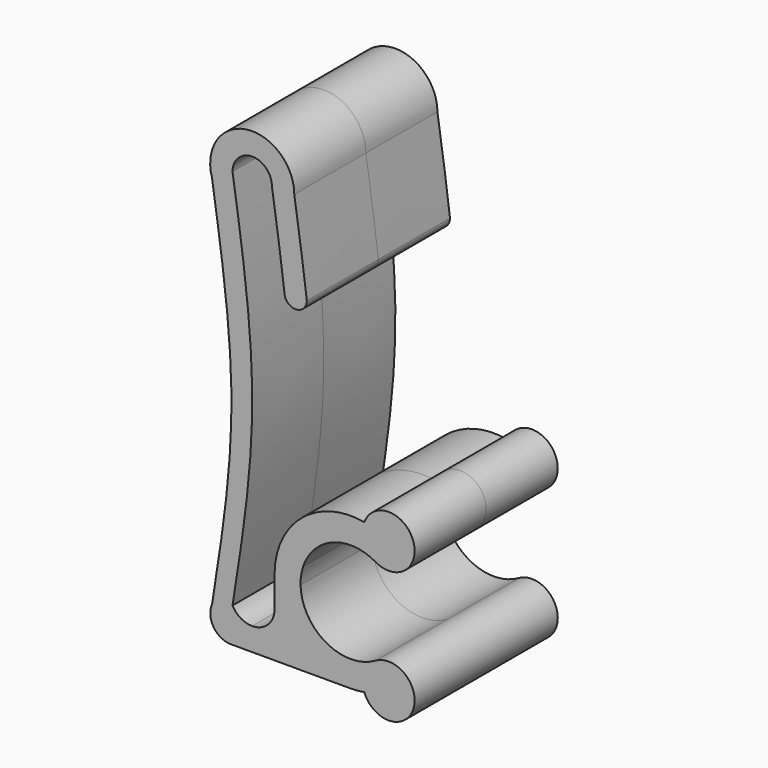
from build123d import *

# Parameters (mm, degrees)
F1_DEPTH = 6.35


# Not quite as in the source:
# - ends of sketch curves that miss each other by under 0.0002 mm in the source are joined
# - the dataset's text gives a spline's control points without its knots; the knots are read off the source's solid


with BuildPart() as f1:
    # F0 (on Front) → F1 (new body, symmetric)
    with BuildSketch(Plane.XZ):
        with BuildLine():
            Line((-8.4141566916, -5.3975), (0, -5.3975))
            ThreePointArc((0, -5.3975), (0.4871232852, -5.375473668), (0.9702708263, -5.3095744437))
            ThreePointArc((0.9702708263, -5.3095744437), (4.4301700946, -5.3015138122), (1.778, -3.0795863359))
            ThreePointArc((1.778, -3.0795863359), (-1.7391660801, -3.101682986), (-3.5548772461, -0.0893519188))
            ThreePointArc((-3.5548772461, -0.0893519188), (-3.5177568499, 0.5201180106), (-3.3769182629, 1.1142526848))
            add(Edge.make_bspline(
                [(-3.3769182629, 1.1142526848), (-3.213886893, 2.2483634663), (-3.0651248799, 3.384623456), (-2.942596945, 4.524834745)],
                knots=[0.1529319216, 0.1529319216, 0.1529319216, 0.1529319216, 0.2811638974, 0.2811638974, 0.2811638974, 0.2811638974], degree=3))
            ThreePointArc((-2.942596945, 4.524834745), (-3.9835985246, 3.6419704892), (-4.7698383359, 2.5261924906))
            add(Edge.make_bspline(
                [(-5.3975, -1.7347033349), (-5.173779235, -0.3165887052), (-4.9567128934, 1.1025281941), (-4.7698383359, 2.5261924906)],
                knots=[0.0454256059, 0.0454256059, 0.0454256059, 0.0454256059, 0.2061005135, 0.2061005135, 0.2061005135, 0.2061005135], degree=3))
            Line((-5.3975, -1.7347033349), (-5.3975, -2.1827106738))
            ThreePointArc((-5.3975, -2.1827106738), (-5.4459433862, -2.5718905674), (-5.5883169948, -2.9373184082))
            ThreePointArc((-5.5883169948, -2.9373184082), (-6.1719143737, -3.5461797839), (-6.985, -3.7702106738))
            ThreePointArc((-6.985, -3.7702106738), (-7.7980896495, -3.5461803993), (-8.3816869181, -2.9373205224))
            add(Edge.make_bspline(
                [(-8.3816869181, -2.9373205224), (-7.6903162591, 1.4077055077), (-6.2862259108, 10.2319288559), (-7.676155344, 19.4769791983), (-8.3816869181, 24.1697893262)],
                knots=[0, 0, 0, 0, 0.4923975582, 1, 1, 1, 1], degree=3))
            ThreePointArc((-8.3816869181, 24.1697893262), (-6.985, 25.5664762444), (-5.5883130819, 24.1697893263))
            add(Edge.make_bspline(
                [(-4.676452861, 17.6339959576), (-4.9321460197, 19.8053249313), (-5.2602295508, 21.9875571288), (-5.5883130819, 24.1697893263)],
                knots=[0.7639566994, 0.7639566994, 0.7639566994, 0.7639566994, 1, 1, 1, 1], degree=3))
            ThreePointArc((-4.676452861, 17.6339959576), (-3.8112048513, 17.0315712658), (-3.1110035111, 17.8197893262))
            add(Edge.make_bspline(
                [(-3.1110035111, 17.8197893262), (-3.3633587069, 19.9297914909), (-3.6820858944, 22.0497904085), (-4.0008130819, 24.1697893262)],
                knots=[0.7706882235, 0.7706882235, 0.7706882235, 0.7706882235, 1, 1, 1, 1], degree=3))
            ThreePointArc((-4.0008130819, 24.1697893262), (-7.4285431353, 27.1208299985), (-9.837338265, 23.292556185))
            add(Edge.make_bspline(
                [(-9.8352581181, -3.3290753137), (-9.6597468246, -2.2260473952), (-9.3104483349, -0.0304942675), (-8.8571977057, 3.2414000554), (-8.5914867755, 5.9577245973), (-8.4768185316, 8.1311720824), (-8.4476359431, 9.7599621423), (-8.4814070197, 11.4021639111), (-8.5995564813, 13.6155987531), (-8.8666228021, 16.4200169888), (-9.3175498954, 19.8349473194), (-9.6635970859, 22.1369248922), (-9.837338265, 23.292556185)],
                knots=[0, 0, 0, 0, 0.125, 0.25, 0.375, 0.4375, 0.5, 0.5625, 0.625, 0.75, 0.875, 1, 1, 1, 1], degree=3))
            ThreePointArc((-9.8352581181, -3.3290753137), (-9.7481101941, -4.6955367779), (-8.5725, -5.3975))
            Line((-8.5725, -5.3975), (-8.4141566916, -5.3975))
        make_face()
        with BuildLine():
            ThreePointArc((-8.5725, -5.3975), (-8.4933283458, -5.399633381), (-8.4141566916, -5.3975))
            Line((-8.4141566916, -5.3975), (-8.5725, -5.3975))
        make_face()
        with BuildLine():
            add(Edge.make_bspline(
                [(-3.3769182629, 1.1142526848), (-3.213886893, 2.2483634663), (-3.0651248799, 3.384623456), (-2.942596945, 4.524834745)],
                knots=[0.1529319216, 0.1529319216, 0.1529319216, 0.1529319216, 0.2811638974, 0.2811638974, 0.2811638974, 0.2811638974], degree=3))
            ThreePointArc((-3.3769182629, 1.1142526848), (-1.2667947714, 3.3227047728), (1.778, 3.0795863359))
            ThreePointArc((1.778, 3.0795863359), (4.4301700946, 5.3015138122), (0.9702708263, 5.3095744437))
            ThreePointArc((0.9702708263, 5.3095744437), (-1.0613537009, 5.2921200451), (-2.942596945, 4.524834745))
        make_face()
        with BuildLine():
            add(Edge.make_bspline(
                [(-5.3975, -1.7347033349), (-5.173779235, -0.3165887052), (-4.9567128934, 1.1025281941), (-4.7698383359, 2.5261924906)],
                knots=[0.0454256059, 0.0454256059, 0.0454256059, 0.0454256059, 0.2061005135, 0.2061005135, 0.2061005135, 0.2061005135], degree=3))
            ThreePointArc((-4.7698383359, 2.5261924906), (-5.2382348491, 1.3014998717), (-5.3975, 0))
            Line((-5.3975, 0), (-5.3975, -1.7347033349))
        make_face()
    extrude(amount=F1_DEPTH, both=True)


solid = f1.part
